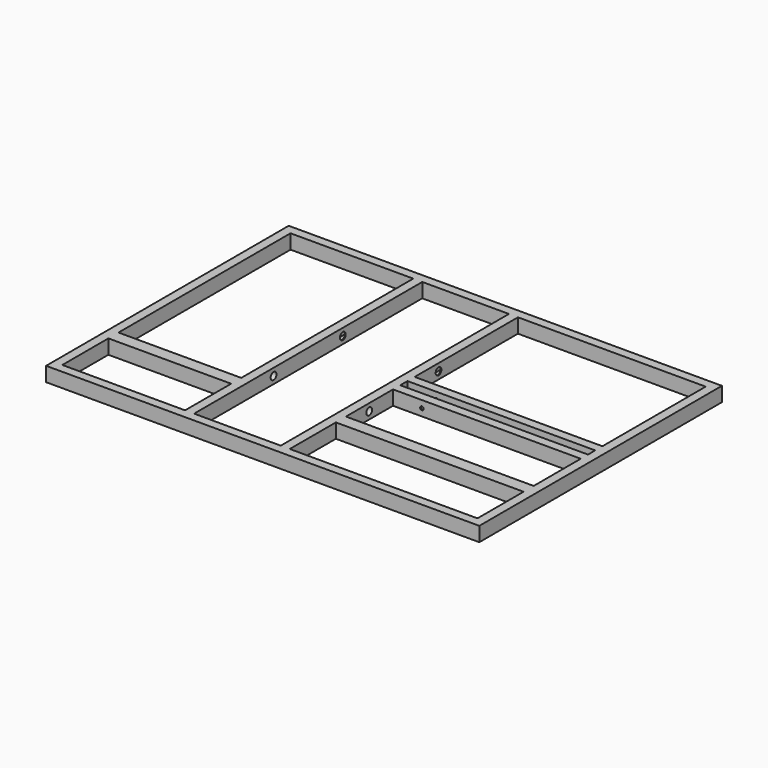
from build123d import *

# Parameters (mm, degrees)
F0_W     = 1524
F0_H     = 1066.8
F0_W_2   = 304.8
F0_H_2   = 1003.3
F0_W_3   = 660.4
F0_H_3   = 31.75
F0_H_4   = 454.025
F0_W_4   = 431.8
F0_H_5   = 44.45
F1_DEPTH = 50.8
F2_R     = 12.7
F3_DEPTH = 406.4
F4_R     = 6.35
F5_DEPTH = 127
F6_T     = -3.175


# Not quite as in the source:
# - a feature names something its author has since deleted; it is built from what else it names


with BuildPart() as f1:
    # F0 (on Top) → F1 (new body)
    with BuildSketch(Plane.XY):
        with Locations((762, -533.4)):
            Rectangle(F0_W, F0_H)
        Polygon((1492.25, -1035.05), (831.85, -1035.05), (831.85, -832.48246), (831.85, -788.03246), (831.85, -581.025), (1492.25, -581.025), (1492.25, -788.03246), (1492.25, -832.48246), align=None, mode=Mode.SUBTRACT)
        Polygon((31.75, -788.03246), (31.75, -31.75), (463.55, -31.75), (463.55, -788.03246), (463.55, -832.48246), (463.55, -1035.05), (31.75, -1035.05), (31.75, -832.48246), align=None, mode=Mode.SUBTRACT)
        with Locations((647.7, -533.4)):
            Rectangle(F0_W_2, F0_H_2, mode=Mode.SUBTRACT)
        with Locations((1162.05, -533.4)):
            Rectangle(F0_W_3, F0_H_3, mode=Mode.SUBTRACT)
        with Locations((1162.05, -258.7625)):
            Rectangle(F0_W_3, F0_H_4, mode=Mode.SUBTRACT)
        with Locations((247.65, -810.25746)):
            Rectangle(F0_W_4, F0_H_5)
        with Locations((1162.05, -810.25746)):
            Rectangle(F0_W_3, F0_H_5)
    extrude(amount=F1_DEPTH)

    # F2 (on face) → F3 (cut)
    with BuildSketch(Plane(origin=(463.55, 0, 0), x_dir=(0, -1, 0), z_dir=(-1, 0, 0))):
        with Locations((381, 25.4)):
            Circle(F2_R)
        with Locations((685.8, 25.4)):
            Circle(F2_R)
    extrude(amount=-F3_DEPTH, mode=Mode.SUBTRACT)

    # F4 (on face) → F5 (cut)
    with BuildSketch(Plane(origin=(0, -485.775, 0), x_dir=(-1, 0, 0), z_dir=(0, 1, 0))):
        with Locations((-933.45, 25.4)):
            Circle(F4_R)
    extrude(amount=-F5_DEPTH, mode=Mode.SUBTRACT)

    # F6
    f6_openings = [f1.faces().sort_by_distance(p)[0] for p in [
        (815.975, -368.3, 25.4),
        (479.425, -368.3, 25.4),
        (939.8, -565.15, 25.4),
        (939.8, -501.65, 25.4),
    ]]
    offset(amount=F6_T, openings=f6_openings, kind=Kind.INTERSECTION)


solid = f1.part
